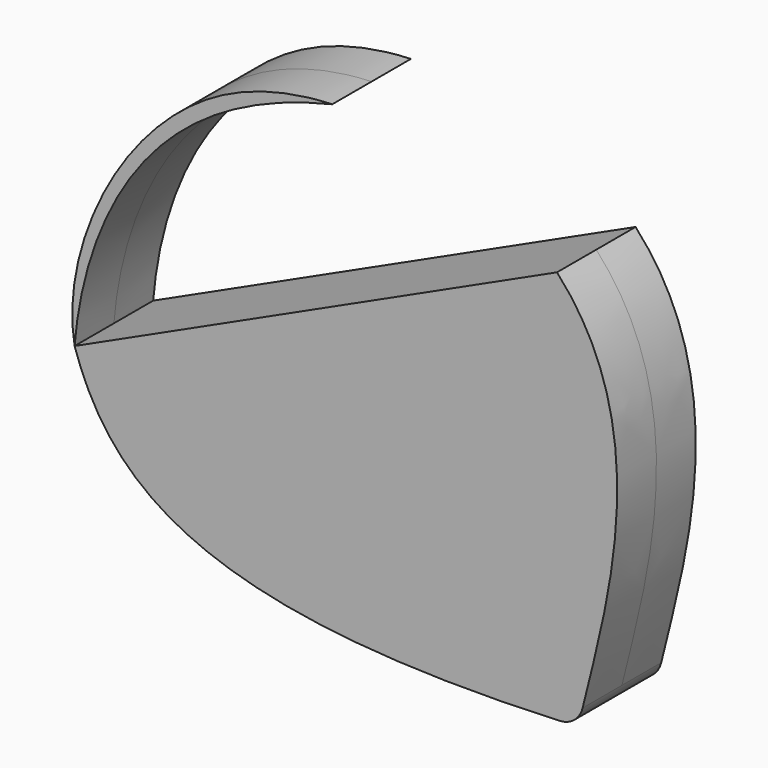
from build123d import *

# Parameters (mm, degrees)
F1_DEPTH = 12.7


with BuildPart() as f1:
    # F0 (on Front) → F1 (new body, symmetric)
    with BuildSketch(Plane.XZ):
        with BuildLine():
            add(Edge.make_bspline(
                [(57.1871035576, 33.0515832115), (83.4640090894, 4.7482788241), (69.8356338221, -39.121123681), (63.8103867226, -63.9335548477)],
                knots=[0, 0, 0, 0, 95.5050447095, 95.5050447095, 95.5050447095, 95.5050447095], degree=3))
            Line((57.1871035576, 33.0515832115), (-67.5041534908, -24.2631812721))
            add(Edge.make_bspline(
                [(57.9210074343, -68.7788861237), (-33.1218832719, -72.8158713516), (-57.8737772663, -53.6331943002), (-67.5041534908, -24.2631812721)],
                knots=[2.3552403512, 2.3552403512, 2.3552403512, 2.3552403512, 137.5659066611, 137.5659066611, 137.5659066611, 137.5659066611], degree=3))
            ThreePointArc((57.9210074343, -68.7788861237), (61.6741008128, -67.3388150573), (63.8103867226, -63.9335548477))
        make_face()
    extrude(amount=F1_DEPTH, both=True)


with BuildPart() as f1b:
    # F0 (on Front) → F1, piece 2 (new body, symmetric)
    with BuildSketch(Plane.XZ):
        with BuildLine():
            add(Edge.make_bspline(
                [(-0.8981807459, 52.4018313512), (-11.0166847084, 50.0759443022), (-54.3602010989, 33.3948801257), (-65.879063599, -3.8987406946), (-67.5041534908, -24.2631812721)],
                knots=[0.3733611821, 0.3733611821, 0.3733611821, 0.3733611821, 0.5164799744, 1, 1, 1, 1], degree=3))
            add(Edge.make_bspline(
                [(-67.5041534908, -24.2631812721), (-71.4835964909, -2.1616155462), (-49.9112308582, 43.0663063494), (-10.8057204253, 52.0165849428), (-0.8981807459, 52.4018313512)],
                knots=[0, 0, 0, 0, 0.488366921, 0.64981559, 0.64981559, 0.64981559, 0.64981559], degree=3))
        make_face()
    extrude(amount=F1_DEPTH, both=True)


solid = Compound([f1.part, f1b.part])
